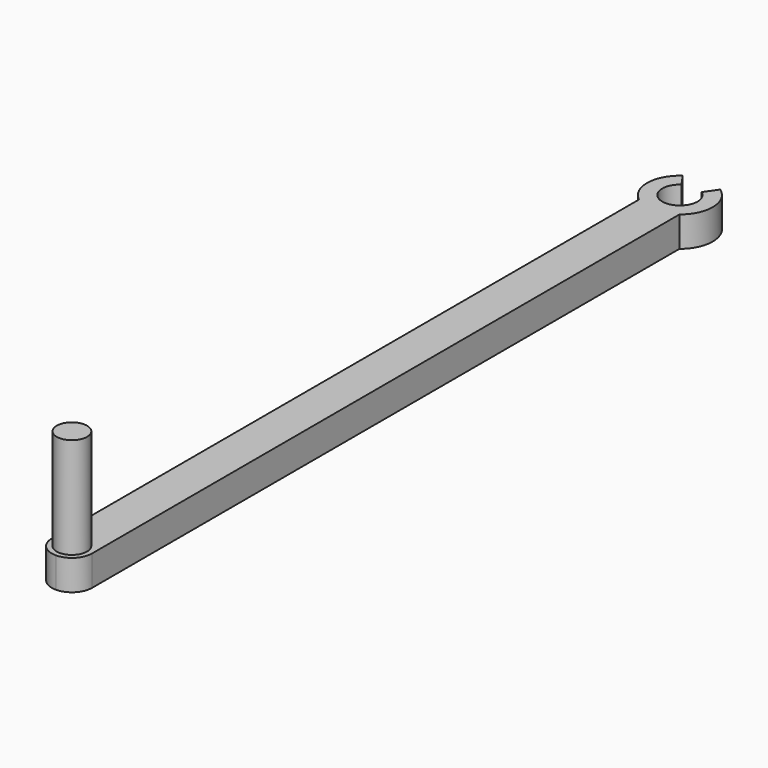
from build123d import *

# Parameters (mm, degrees)
F1_DEPTH = 3
F2_R     = 1.5
F3_DEPTH = 10


# Not quite as in the source:
# - a feature names something its author has since deleted; it is built from what else it names


with BuildPart() as f1:
    # F0 (on Top) → F1 (new body)
    with BuildSketch(Plane.XY):
        with BuildLine():
            ThreePointArc((3.25, 74.9241337907), (2.1924432633, 75.1010126169), (1.25, 75.6123960992))
            Line((1.25, 75.6123960992), (1.25, 2.9241337907))
            ThreePointArc((1.25, 2.9241337907), (1.8357864376, 4.338347353), (3.25, 4.9241337907))
            Line((3.25, 4.9241337907), (3.25, 74.9241337907))
        make_face()
        with BuildLine():
            ThreePointArc((3.25, 4.9241337907), (1.8357864376, 4.338347353), (1.25, 2.9241337907))
            ThreePointArc((1.25, 2.9241337907), (1.8357864376, 1.5099202283), (3.25, 0.9241337907))
            Line((3.25, 0.9241337907), (3.25, 4.9241337907))
        make_face()
        with BuildLine():
            ThreePointArc((5.25, 75.6123960992), (4.3075567367, 75.1010126169), (3.25, 74.9241337907))
            Line((3.25, 74.9241337907), (3.25, 4.9241337907))
            ThreePointArc((3.25, 4.9241337907), (4.6642135624, 4.338347353), (5.25, 2.9241337907))
            Line((5.25, 2.9241337907), (5.25, 75.6123960992))
        make_face()
        with BuildLine():
            ThreePointArc((5.25, 2.9241337907), (4.6642135624, 4.338347353), (3.25, 4.9241337907))
            Line((3.25, 4.9241337907), (3.25, 0.9241337907))
            ThreePointArc((3.25, 0.9241337907), (4.6642135624, 1.5099202283), (5.25, 2.9241337907))
        make_face()
        with BuildLine():
            Line((2.25, 79.6102744523), (1.3928571429, 80.8412521623))
            ThreePointArc((1.3928571429, 80.8412521623), (0.0012122742, 78.2628936507), (1.25, 75.6123960992))
            ThreePointArc((1.25, 75.6123960992), (2.1924432633, 75.1010126169), (3.25, 74.9241337907))
            ThreePointArc((3.25, 74.9241337907), (4.3075567367, 75.1010126169), (5.25, 75.6123960992))
            ThreePointArc((5.25, 75.6123960992), (6.4987877258, 78.2628936507), (5.1071428571, 80.8412521623))
            Line((5.1071428571, 80.8412521623), (4.25, 79.6102744523))
            ThreePointArc((4.25, 79.6102744523), (3.25, 76.4241337907), (2.25, 79.6102744523))
        make_face()
    extrude(amount=F1_DEPTH)

    # F2 (on face) → F3 (join)
    with BuildSketch(Plane.XY.offset(3)):
        with Locations((3.25, 2.9241337907)):
            Circle(F2_R)
    extrude(amount=F3_DEPTH)


solid = f1.part
